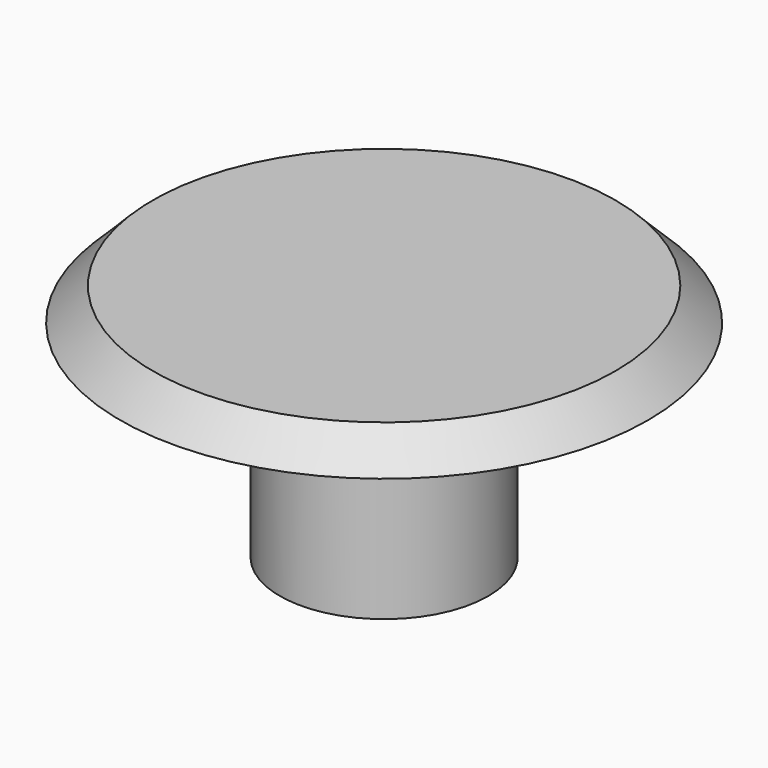
from build123d import *

# Parameters (mm, degrees)
F2_SIZE  = 1.27
F3_R     = 18.9556070846
F3_R_2   = 5.842
F4_DEPTH = 0.8
F5_SIZE  = 1.016


# Not quite as in the source:
# - a fillet or chamfer that OpenCascade refuses, or shapes differently, is made with other operations: its cross-section is extruded or revolved along the edge and cut away or added


with BuildPart() as f1:
    # F0 (on Front) → F1 (revolve)
    with BuildSketch(Plane.XZ):
        with BuildLine():
            Line((0, 0), (2.6757909362, 0))
            Line((2.6757909362, 0), (2.6757909362, -3.438))
            ThreePointArc((2.6757909362, -3.438), (2.2947909362, -3.819), (2.6757909362, -4.2))
            Line((2.6757909362, -4.2), (2.6757909362, -7))
            Line((2.6757909362, -7), (3.937, -7))
            Line((3.937, -7), (3.937, 0))
            Line((3.937, 0), (10, 0))
            Line((10, 0), (10, 2.032))
            Line((10, 2.032), (0, 2.032))
            Line((0, 2.032), (0, 0))
        make_face()
    revolve(axis=Axis((0, 0, 1.016), (0, 0, -1)))

    # F2
    f2_edges = [f1.edges().sort_by_distance(p)[0] for p in [
        (-2.675791, 0, 0),
    ]]
    chamfer(f2_edges, length=F2_SIZE)

    # F3 (on face) → F4 (cut)
    with BuildSketch(Plane(origin=(0, 0, 0), x_dir=(1, 0, 0), z_dir=(0, 0, -1))):
        with Locations((0, -0.8832210264)):
            Circle(F3_R)
        Circle(F3_R_2, mode=Mode.SUBTRACT)
    extrude(amount=-F4_DEPTH, mode=Mode.SUBTRACT)

    # F5
    f5_edges = [f1.edges().sort_by_distance(p)[0] for p in [
        (-2.675791, 0, -7),
    ]]
    chamfer(f5_edges, length=F5_SIZE)

    # F6: chamfer of 1.27 on 1 edges, made by hand

    # F6_s1 → F6_t2 (revolve, cut)
    with BuildSketch(Plane.XZ):
        Polygon((10, 0.762), (8.73, 2.032), (10, 2.032), align=None)
    revolve(axis=Axis((0, 0, 2.032), (0, 0, -1)), mode=Mode.SUBTRACT)


solid = f1.part
